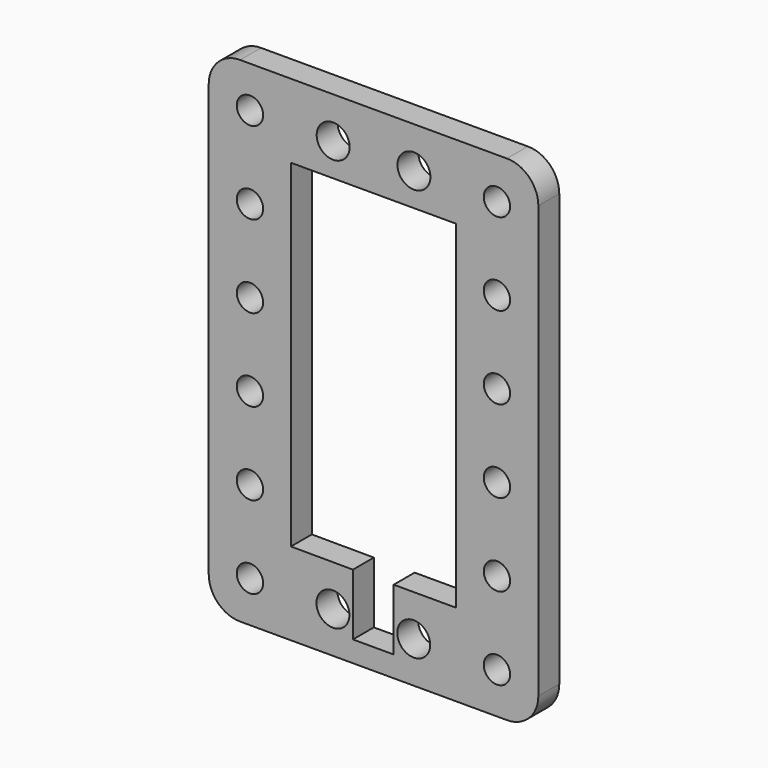
from build123d import *

# Parameters (mm, degrees)
F0_R     = 1.6
F0_R_2   = 2
F1_DEPTH = 3.175


# Not quite as in the source:
# - a length typed as a fraction of an inch, garbled in the dataset ("3 / 203.2 mm" for 3/8 in), is restored


with BuildPart() as f1:
    # F0 (on Front) → F1 (new body)
    with BuildSketch(Plane.XZ):
        with BuildLine():
            Line((26.215, 8.975), (-6.165, 8.975))
            ThreePointArc((-6.165, 8.975), (-8.8590768363, 7.8590768363), (-9.975, 5.165))
            Line((-9.975, 5.165), (-9.975, -47.215))
            ThreePointArc((-9.975, -47.215), (-8.8590768363, -49.9090768363), (-6.165, -51.025))
            Line((-6.165, -51.025), (26.215, -51.025))
            ThreePointArc((26.215, -51.025), (28.9090768363, -49.9090768363), (30.025, -47.215))
            Line((30.025, -47.215), (30.025, 5.165))
            ThreePointArc((30.025, 5.165), (28.9090768363, 7.8590768363), (26.215, 8.975))
        make_face()
        with Locations((-4.975, -46.025)):
            Circle(F0_R, mode=Mode.SUBTRACT)
        with Locations((5.1, -46.025)):
            Circle(F0_R_2, mode=Mode.SUBTRACT)
        with Locations((-4.975, -36.025)):
            Circle(F0_R, mode=Mode.SUBTRACT)
        with Locations((-4.975, -26.025)):
            Circle(F0_R, mode=Mode.SUBTRACT)
        Polygon((0, -41), (0, 0), (20.025, 0), (20.025, -41.025), (12.4728614733, -41.025), (12.4728614733, -48.485), (7.5228614733, -48.485), (7.5228614733, -41.025), align=None, mode=Mode.SUBTRACT)
        with Locations((14.9, -46.025)):
            Circle(F0_R_2, mode=Mode.SUBTRACT)
        with Locations((25, -46.025)):
            Circle(F0_R, mode=Mode.SUBTRACT)
        with Locations((25, -36.025)):
            Circle(F0_R, mode=Mode.SUBTRACT)
        with Locations((25, -26.025)):
            Circle(F0_R, mode=Mode.SUBTRACT)
        with Locations((-4.975, -16.025)):
            Circle(F0_R, mode=Mode.SUBTRACT)
        with Locations((-4.975, -6.025)):
            Circle(F0_R, mode=Mode.SUBTRACT)
        with Locations((-4.975, 3.975)):
            Circle(F0_R, mode=Mode.SUBTRACT)
        with Locations((5.125, 3.975)):
            Circle(F0_R_2, mode=Mode.SUBTRACT)
        with Locations((25, -16.025)):
            Circle(F0_R, mode=Mode.SUBTRACT)
        with Locations((14.925, 3.975)):
            Circle(F0_R_2, mode=Mode.SUBTRACT)
        with Locations((25, -6.025)):
            Circle(F0_R, mode=Mode.SUBTRACT)
        with Locations((25, 3.975)):
            Circle(F0_R, mode=Mode.SUBTRACT)
    extrude(amount=F1_DEPTH)


solid = f1.part
